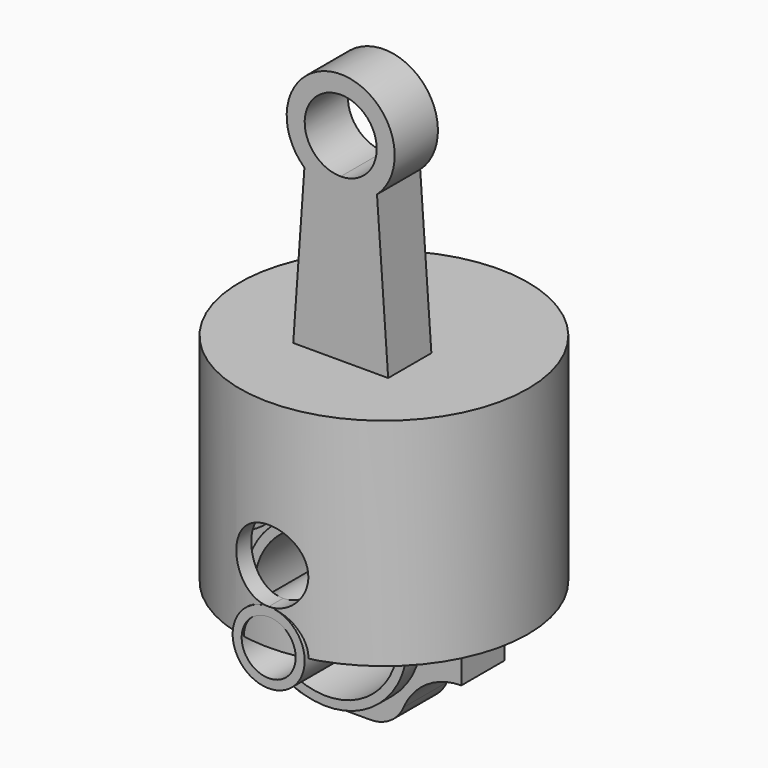
from build123d import *

# Parameters (mm, degrees)
F1_DEPTH       = 19.05
F2_R           = 28.575
F2_R_2         = 25.4
F3_DEPTH       = 25.4
F4_R           = 28.575
F4_R_2         = 25.4
F5_DEPTH       = 6.35
F6_R           = 12.7
F7_R           = 6.35
F8_R           = 12.7
F8_R_2         = 9.525
F9_DEPTH       = 50.8
F9_DEPTH_BACK  = 50.8
F10_R          = 50.8
F10_R_2        = 44.45
F11_DEPTH      = 76.2
F12_R          = 50.8
F13_DEPTH      = 12.7
F15_DEPTH      = 72.136
F15_DEPTH_BACK = 101.346


with BuildPart() as f1:
    # F0 (on Front) → F1 (new body)
    with BuildSketch(Plane.XZ):
        with BuildLine():
            Line((-12.7996388564, 131.9407213102), (-20.4085066075, 24.321911069))
            ThreePointArc((-20.4085066075, 24.321911069), (-29.5849648539, 14.4892969079), (-42.53524071, 10.8591395506))
            Line((-42.53524071, 10.8591395506), (-42.53524071, -10.8591395506))
            ThreePointArc((-42.53524071, -10.8591395506), (-27.2539153671, -16.9737049796), (-20.4085066075, -31.941911069))
            Line((-20.4085066075, -31.941911069), (20.4085066075, -31.941911069))
            ThreePointArc((20.4085066075, -31.941911069), (27.2539153671, -16.9737049796), (42.53524071, -10.8591395506))
            Line((42.53524071, -10.8591395506), (42.53524071, 10.8591395506))
            ThreePointArc((42.53524071, 10.8591395506), (29.5849648539, 14.4892969079), (20.4085066075, 24.321911069))
            Line((20.4085066075, 24.321911069), (12.7996388564, 131.9407213102))
            ThreePointArc((12.7996388564, 131.9407213102), (0, 165.1), (-12.7996388564, 131.9407213102))
        make_face()
        with BuildLine():
            ThreePointArc((0, -28.575), (-20.2055762724, 20.2055762724), (28.575, 0))
            ThreePointArc((28.575, 0), (20.2055762724, -20.2055762724), (0, -28.575))
        make_face(mode=Mode.SUBTRACT)
        with BuildLine():
            ThreePointArc((0, 133.35), (-8.9802561211, 155.0302561211), (12.7, 146.05))
            ThreePointArc((12.7, 146.05), (8.9802561211, 137.0697438789), (0, 133.35))
        make_face(mode=Mode.SUBTRACT)
    extrude(amount=F1_DEPTH)

    # F2 (on Front) → F3 (join)
    with BuildSketch(Plane.XZ):
        Circle(F2_R)
        Circle(F2_R_2, mode=Mode.SUBTRACT)
    extrude(amount=F3_DEPTH)

    # F4 (on face) → F5 (join)
    with BuildSketch(Plane(origin=(0, 0, 0), x_dir=(-1, 0, 0), z_dir=(0, 1, 0))):
        Circle(F4_R)
        Circle(F4_R_2, mode=Mode.SUBTRACT)
    extrude(amount=F5_DEPTH)

    # F6
    f6_edges = [f1.edges().sort_by_distance(p)[0] for p in [
        (20.408507, -9.525, -31.941911),
        (-20.408507, -9.525, -31.941911),
    ]]
    fillet(f6_edges, radius=F6_R)

    # F7
    f7_edges = [f1.edges().sort_by_distance(p)[0] for p in [
        (42.535241, -9.525, 10.85914),
        (-42.535241, -9.525, 10.85914),
    ]]
    fillet(f7_edges, radius=F7_R)


with BuildPart() as f9:
    # F8 (on Front) → F9 (new body, two sides)
    with BuildSketch(Plane.XZ) as f9_sk:
        Circle(F8_R)
        Circle(F8_R_2, mode=Mode.SUBTRACT)
    extrude(amount=F9_DEPTH)
    extrude(f9_sk.sketch, amount=-F9_DEPTH_BACK)


with BuildPart() as f11:
    # F10 (on Top) → F11 (new body)
    with BuildSketch(Plane.XY):
        Circle(F10_R)
        Circle(F10_R_2, mode=Mode.SUBTRACT)
    extrude(amount=F11_DEPTH)

    # F12 (on face) → F13 (join)
    with BuildSketch(Plane.XY.offset(76.2)):
        Circle(F12_R)
    extrude(amount=-F13_DEPTH)

    # F14 (on Front) → F15 (cut, two sides)
    with BuildSketch(Plane.XZ) as f15_sk:
        with BuildLine():
            ThreePointArc((0, 12.7), (8.9802561211, 16.4197438789), (12.7, 25.4))
            ThreePointArc((12.7, 25.4), (-8.9802561211, 34.3802561211), (0, 12.7))
        make_face()
    extrude(amount=-F15_DEPTH, mode=Mode.SUBTRACT)
    extrude(f15_sk.sketch, amount=F15_DEPTH_BACK, mode=Mode.SUBTRACT)


solid = Compound([f1.part, f9.part, f11.part])
